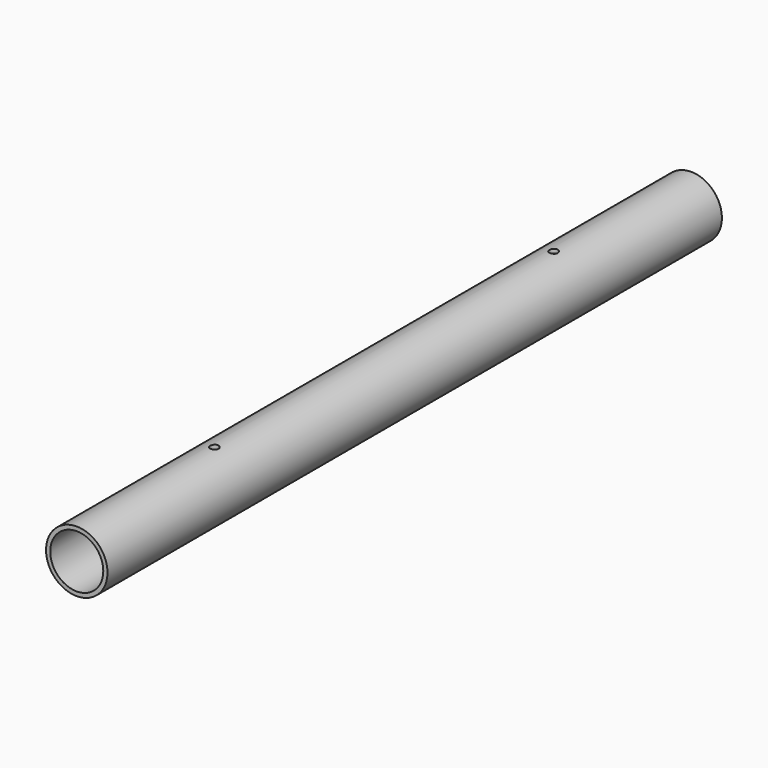
from build123d import *

# Parameters (mm, degrees)
F0_R     = 11
F0_R_2   = 9.5
F1_DEPTH = 137.5
F2_R     = 1.5
F3_DEPTH = 12.5


# Not quite as in the source:
# - a pattern or mirror of a feature is missing from the dataset's text; its kind, count and spacing are read off the source's solid


with BuildPart() as f1:
    # F0 (on Front) → F1 (new body, symmetric)
    with BuildSketch(Plane.XZ):
        Circle(F0_R)
        Circle(F0_R_2, mode=Mode.SUBTRACT)
    extrude(amount=F1_DEPTH, both=True)

    # F2 (on Top) → F3 (cut, symmetric)
    with BuildSketch(Plane.XY):
        with Locations((0, -75.9)):
            Circle(F2_R)
    f3 = extrude(amount=F3_DEPTH, both=True, mode=Mode.SUBTRACT)

    # F3_copies: F3 across plane
    add(f3.mirror(Plane.ZX.offset(2e-06)), mode=Mode.SUBTRACT)


solid = f1.part
